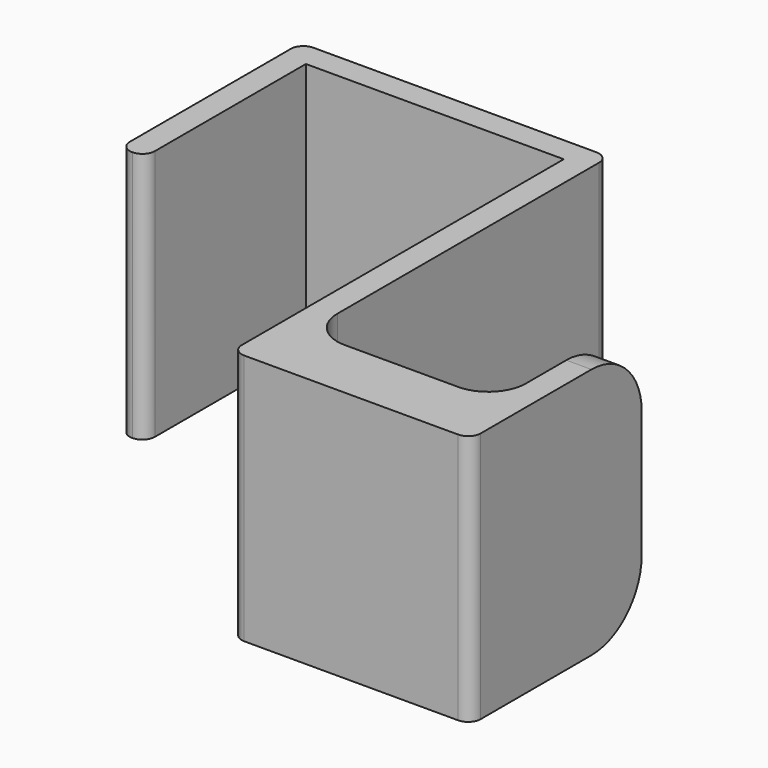
from build123d import *

# Parameters (mm, degrees)
F1_DEPTH = 20
F2_R     = 5
F3_R     = 0.99999
F4_R     = 3


# Not quite as in the source:
# - a fillet or chamfer is up to 0.001 mm smaller than in the source, because OpenCascade refuses the exact size


with BuildPart() as f1:
    # F0 (on Top) → F1 (new body)
    with BuildSketch(Plane.XY):
        Polygon((0, 18), (0, 0), (2, 0), (2, 16), (22.5, 16), (22.5, -17), (41.5, -17), (41.5, 0), (39.5, 0), (39.5, -12), (24.5, -12), (24.5, 18), align=None)
    extrude(amount=F1_DEPTH)

    # F2
    f2_edges = [f1.edges().sort_by_distance(p)[0] for p in [
        (40.5, 0, 20),
        (40.5, 0, 0),
    ]]
    fillet(f2_edges, radius=F2_R)

    # F3 (radius 1 in the source; OpenCascade refuses exactly that, so slightly less here)
    f3_edges = [f1.edges().sort_by_distance(p)[0] for p in [
        (0, 18, 10),
        (24.5, 18, 10),
        (2, 0, 10),
        (22.5, -17, 10),
        (41.5, -17, 10),
        (0, 0, 10),
    ]]
    fillet(f3_edges, radius=F3_R)

    # F4
    f4_edges = [f1.edges().sort_by_distance(p)[0] for p in [
        (24.5, -12, 10),
        (39.5, -12, 10),
    ]]
    fillet(f4_edges, radius=F4_R)


solid = f1.part
